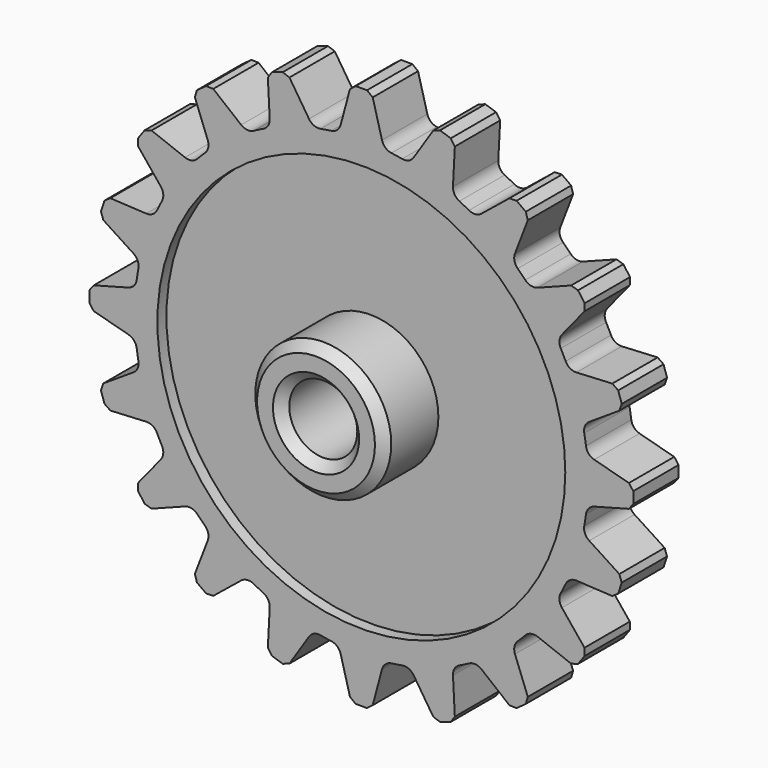
from build123d import *

# Parameters (mm, degrees)
F0_R            = 100
F1_DEPTH        = 25
F3_DEPTH        = 25
F3_COPIES_COUNT = 20
F4_SIZE         = 2
F5_R            = 5
F6_R            = 90
F7_DEPTH        = 5
F8_R            = 30
F9_DEPTH        = 30
F10_R           = 15
F11_DEPTH       = 50.001
F12_SIZE        = 4


# Not quite as in the source:
# - a pattern or mirror of a feature is missing from the dataset's text; its kind, count and spacing are read off the source's solid


with BuildPart() as f1:
    # F0 (on Front) → F1 (new body)
    with BuildSketch(Plane.XZ):
        Circle(F0_R)
    extrude(amount=F1_DEPTH)

    # F2 (on face) → F3 (join)
    with BuildSketch(Plane.XZ.offset(25)):
        with BuildLine():
            ThreePointArc((100, 0), (74.159662072, 67.0846071865), (9.9931095726, 99.4994359837))
            Line((9.9931095726, 99.4994359837), (-9.9931095726, 99.4994359837))
            ThreePointArc((-9.9931095726, 99.4994359837), (-67.0846071865, -74.159662072), (100, 0))
        make_face()
        with BuildLine():
            Line((9.9931095726, 99.4994359837), (4.5, 120))
            Line((4.5, 120), (-4.5, 120))
            Line((-4.5, 120), (-9.9931095726, 99.4994359837))
            ThreePointArc((-9.9931095726, 99.4994359837), (0, 100), (9.9931095726, 99.4994359837))
        make_face()
    f3 = extrude(amount=-F3_DEPTH)

    # F3_copies: F3 ×20 about axis
    f3_copies_axis = Axis((0, 0, 0), (0, 1, 0))
    for i in range(1, F3_COPIES_COUNT):
        add(f3.rotate(f3_copies_axis, i * 360 / F3_COPIES_COUNT))

    # F4
    f4_edges = [f1.edges().sort_by_distance(p)[0] for p in [
        (-4.5, -12.5, 120),
        (4.5, -12.5, 120),
        (-41.361794, -12.5, 112.736205),
        (-66.893654, -12.5, 99.727073),
        (-32.802285, -12.5, 115.517358),
        (-74.174807, -12.5, 94.437006),
        (32.802285, -12.5, 115.517358),
        (41.361794, -12.5, 112.736205),
        (66.893654, -12.5, 99.727073),
        (74.174807, -12.5, 94.437006),
        (94.437006, -12.5, 74.174807),
        (99.727073, -12.5, 66.893654),
        (112.736205, -12.5, 41.361794),
        (115.517358, -12.5, 32.802285),
        (120, -12.5, 4.5),
        (120, -12.5, -4.5),
        (115.517358, -12.5, -32.802285),
        (112.736205, -12.5, -41.361794),
        (99.727073, -12.5, -66.893654),
        (94.437006, -12.5, -74.174807),
        (74.174807, -12.5, -94.437006),
        (66.893654, -12.5, -99.727073),
        (41.361794, -12.5, -112.736205),
        (32.802285, -12.5, -115.517358),
        (4.5, -12.5, -120),
        (-4.5, -12.5, -120),
        (-32.802285, -12.5, -115.517358),
        (-41.361794, -12.5, -112.736205),
        (-66.893654, -12.5, -99.727073),
        (-74.174807, -12.5, -94.437006),
        (-94.437006, -12.5, -74.174807),
        (-99.727073, -12.5, -66.893654),
        (-112.736205, -12.5, -41.361794),
        (-115.517358, -12.5, -32.802285),
        (-120, -12.5, -4.5),
        (-120, -12.5, 4.5),
        (-115.517358, -12.5, 32.802285),
        (-112.736205, -12.5, 41.361794),
        (-99.727073, -12.5, 66.893654),
        (-94.437006, -12.5, 74.174807),
    ]]
    chamfer(f4_edges, length=F4_SIZE)

    # F5
    f5_edges = [f1.edges().sort_by_distance(p)[0] for p in [
        (9.99311, -12.5, 99.499436),
        (-9.99311, -12.5, 99.499436),
        (21.243005, -12.5, 97.717628),
        (-21.243005, -12.5, 97.717628),
        (40.251029, -12.5, 91.541546),
        (50.399706, -12.5, 86.370537),
        (-40.251029, -12.5, 91.541546),
        (-50.399706, -12.5, 86.370537),
        (66.568897, -12.5, 74.622932),
        (74.622932, -12.5, 66.568897),
        (-66.568897, -12.5, 74.622932),
        (-74.622932, -12.5, 66.568897),
        (86.370537, -12.5, 50.399706),
        (91.541546, -12.5, 40.251029),
        (-86.370537, -12.5, 50.399706),
        (-91.541546, -12.5, 40.251029),
        (97.717628, -12.5, 21.243005),
        (99.499436, -12.5, 9.99311),
        (-97.717628, -12.5, 21.243005),
        (-99.499436, -12.5, 9.99311),
        (99.499436, -12.5, -9.99311),
        (97.717628, -12.5, -21.243005),
        (-99.499436, -12.5, -9.99311),
        (-97.717628, -12.5, -21.243005),
        (91.541546, -12.5, -40.251029),
        (86.370537, -12.5, -50.399706),
        (-91.541546, -12.5, -40.251029),
        (-86.370537, -12.5, -50.399706),
        (74.622932, -12.5, -66.568897),
        (66.568897, -12.5, -74.622932),
        (-74.622932, -12.5, -66.568897),
        (-66.568897, -12.5, -74.622932),
        (50.399706, -12.5, -86.370537),
        (40.251029, -12.5, -91.541546),
        (-50.399706, -12.5, -86.370537),
        (-40.251029, -12.5, -91.541546),
        (21.243005, -12.5, -97.717628),
        (9.99311, -12.5, -99.499436),
        (-21.243005, -12.5, -97.717628),
        (-9.99311, -12.5, -99.499436),
    ]]
    fillet(f5_edges, radius=F5_R)

    # F6 (on face) → F7 (cut)
    with BuildSketch(Plane.XZ.offset(25)):
        Circle(F6_R)
    extrude(amount=-F7_DEPTH, mode=Mode.SUBTRACT)

    # F8 (on face) → F9 (join)
    with BuildSketch(Plane.XZ.offset(20)):
        Circle(F8_R)
    extrude(amount=F9_DEPTH)

    # F10 (on face) → F11 (cut, through all)
    with BuildSketch(Plane.XZ.offset(50)):
        Circle(F10_R)
    extrude(amount=-F11_DEPTH, mode=Mode.SUBTRACT)

    # F12
    f12_edges = [f1.edges().sort_by_distance(p)[0] for p in [
        (-15, -50, 0),
        (15, -25, 0),
        (-15, 0, 0),
        (-30, -50, 0),
    ]]
    chamfer(f12_edges, length=F12_SIZE)


solid = f1.part
